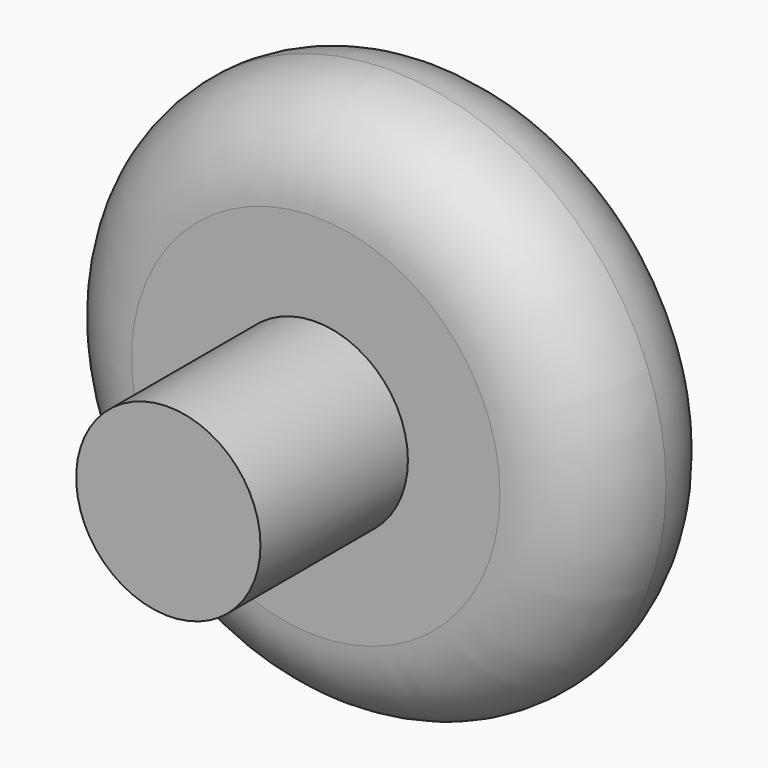
from build123d import *

# Parameters (mm, degrees)
F0_R     = 15
F1_DEPTH = 10
F2_R     = 5
F3_DEPTH = 10
F4_R     = 5
F5_R     = 4.99999


# Not quite as in the source:
# - a fillet or chamfer is up to 0.001 mm smaller than in the source, because OpenCascade refuses the exact size


with BuildPart() as f1:
    # F0 (on Front) → F1 (new body)
    with BuildSketch(Plane.XZ):
        Circle(F0_R)
    extrude(amount=-F1_DEPTH)

    # F2 (on face) → F3 (join)
    with BuildSketch(Plane.XZ):
        Circle(F2_R)
    extrude(amount=F3_DEPTH)

    # F4
    f4_edges = [f1.edges().sort_by_distance(p)[0] for p in [
        (-15, 10, 0),
    ]]
    fillet(f4_edges, radius=F4_R)

    # F5 (radius 5 in the source; OpenCascade refuses exactly that, so slightly less here)
    f5_edges = [f1.edges().sort_by_distance(p)[0] for p in [
        (-15, 0, 0),
    ]]
    fillet(f5_edges, radius=F5_R)


solid = f1.part
